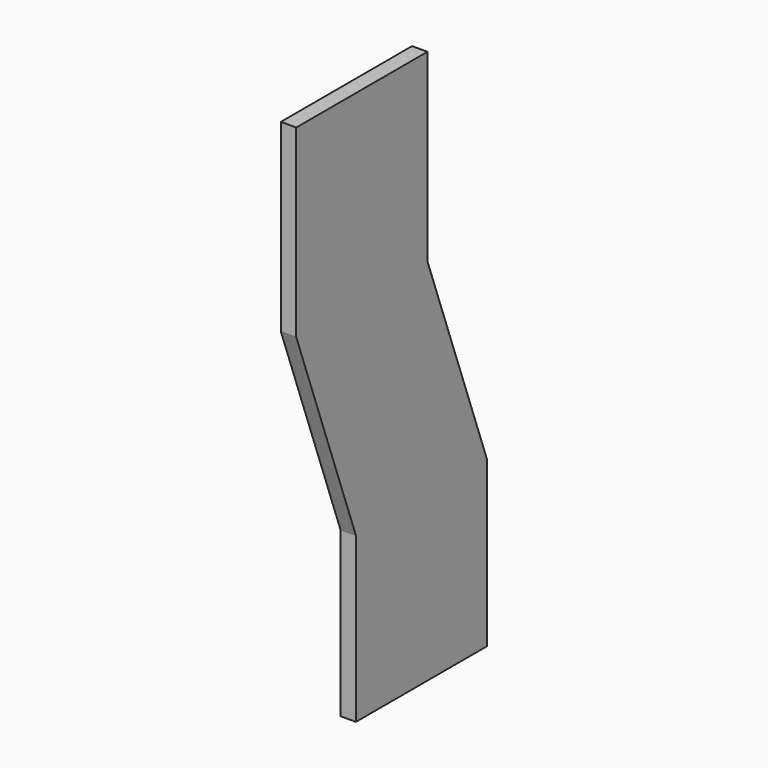
from build123d import *

# Parameters (mm, degrees)
F1_DEPTH = 4.7625


# Not quite as in the source:
# - a feature names something its author has since deleted; it is built from what else it names


with BuildPart() as f1:
    # F0 (on Right) → F1 (new body)
    with BuildSketch(Plane.YZ):
        Polygon((-48.5121098759, 114.3), (-25.4, 50.8), (-25.4, 0), (25.4, 0), (25.4, 50.8), (2.2878901241, 114.3), (2.2878901241, 171.45), (-48.5121098759, 171.45), align=None)
    extrude(amount=F1_DEPTH)


solid = f1.part
